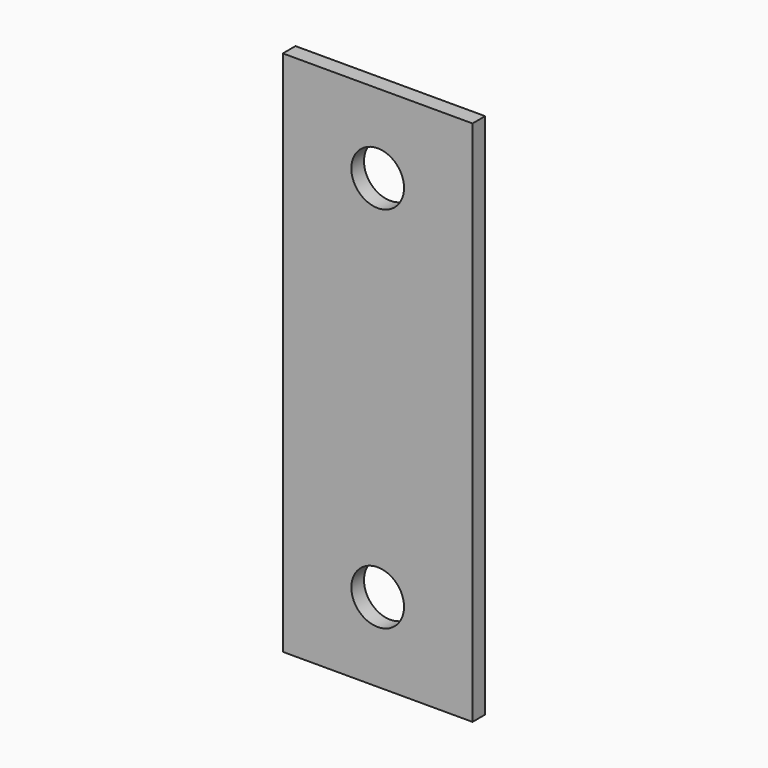
from build123d import *

# Parameters (mm, degrees)
F0_W     = 18
F0_H     = 50
F0_R     = 2.5
F1_DEPTH = 1.5


# Not quite as in the source:
# - a feature names something its author has since deleted; it is built from what else it names


with BuildPart() as f1:
    # F0 (on Front) → F1 (new body)
    with BuildSketch(Plane.XZ):
        with Locations((-9, 25)):
            Rectangle(F0_W, F0_H)
        with Locations((-9, 7.5)):
            Circle(F0_R, mode=Mode.SUBTRACT)
        with Locations((-9, 42.5)):
            Circle(F0_R, mode=Mode.SUBTRACT)
    extrude(amount=F1_DEPTH)


solid = f1.part
